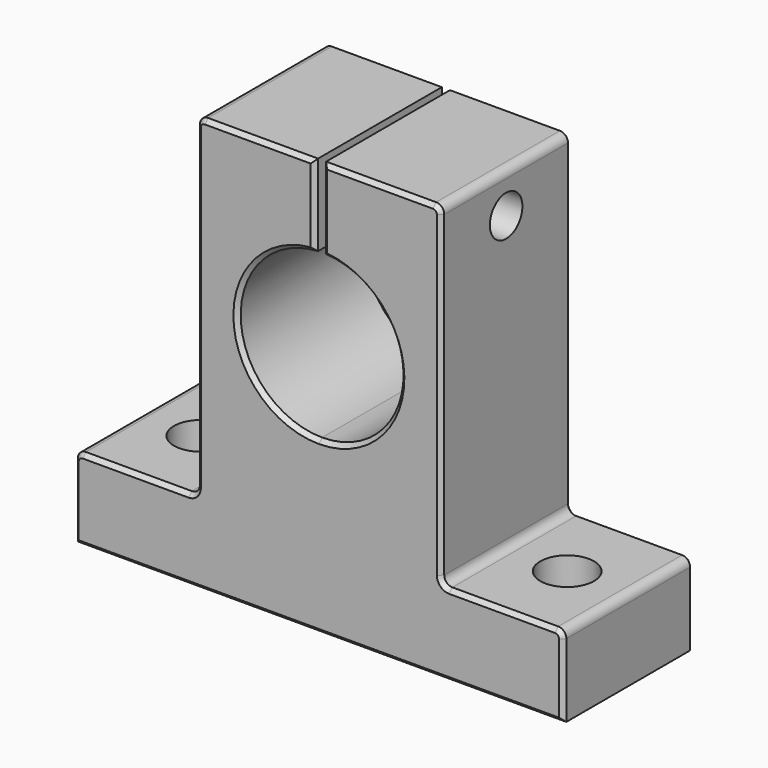
from build123d import *

# Parameters (mm, degrees)
F1_DEPTH    = 10
F3_D        = 6.6
F6_D        = 5
F6_DEPTH    = 22
F6_TIP      = 1.5021515476
F7_R        = 1
F8_C1_SIZE  = 0.5
F8_C2_SIZE  = 0.5
F8_C3_SIZE  = 0.5
F8_C4_SIZE  = 0.5
F8_C5_SIZE  = 0.5
F8_C6_SIZE  = 0.5
F8_C7_SIZE  = 0.5
F8_C8_SIZE  = 0.5
F8_C9_SIZE  = 0.5
F8_C10_SIZE = 0.5
F8_C11_SIZE = 0.5
F8_C12_SIZE = 0.5


with BuildPart() as f1:
    # F0 (on Front) → F1 (new body, symmetric)
    with BuildSketch(Plane.XZ):
        with BuildLine():
            Line((15, 51), (0.5, 51))
            Line((0.5, 51), (0.5, 40.9874921777))
            ThreePointArc((0.5, 40.9874921777), (9.9968725554, 30.7499217894), (0, 21))
            Line((0, 21), (0, 0))
            Line((0, 0), (30, 0))
            Line((30, 0), (30, 10))
            Line((30, 10), (15, 10))
            Line((15, 10), (15, 51))
        make_face()
    extrude(amount=F1_DEPTH, both=True)

    # F3 (through all)
    with Locations(Plane(origin=(0, 0, 0), x_dir=(1, 0, 0), z_dir=(0, 0, -1))):
        with Locations((22.5, 0)):
            Hole(F3_D / 2)

    # F4: F1 across plane


with BuildPart() as f1_1:
    add(f1.part)
    add(f1.part.mirror(Plane.YZ))

    # F6
    with Locations(Plane.YZ.offset(15)):
        with Locations((0, 46)):
            Hole(F6_D / 2, depth=F6_DEPTH)
            with Locations((0, 0, -(F6_DEPTH + F6_TIP / 2))):  # 118° drill point
                Cone(0, F6_D / 2, F6_TIP, mode=Mode.SUBTRACT)

    # F7
    f7_edges = [f1_1.edges().sort_by_distance(p)[0] for p in [
        (15, 0, 10),
        (-15, 0, 10),
        (-30, 0, 10),
        (30, 0, 10),
        (15, 0, 51),
        (-15, 0, 51),
    ]]
    fillet(f7_edges, radius=F7_R)

    # F8: chamfer of 0.5 on 36 edges, made by hand

    # F8_c1
    f8_c1_edges = [f1_1.edges().sort_by_distance(p)[0] for p in [
        (30, 10, 4.5),
        (29.7071067812, 10, 9.7071067812),
        (22.5, 10, 10),
        (15.2928932188, 10, 10.2928932188),
        (15, 10, 30.5),
        (14.7071067812, 10, 50.7071067812),
        (7.25, 10, 51),
    ]]
    chamfer(f8_c1_edges, length=F8_C1_SIZE)

    # F8_c2
    f8_c2_edges = [f1_1.edges().sort_by_distance(p)[0] for p in [
        (-0.25, 10, 0),
    ]]
    chamfer(f8_c2_edges, length=F8_C2_SIZE)

    # F8_c3
    f8_c3_edges = [f1_1.edges().sort_by_distance(p)[0] for p in [
        (-30, 10, 4.75),
        (-29.7071067812, 10, 9.7071067812),
        (-22.5, 10, 10),
        (-15.2928932188, 10, 10.2928932188),
        (-15, 10, 30.5),
        (-14.7071067812, 10, 50.7071067812),
        (-7.25, 10, 51),
    ]]
    chamfer(f8_c3_edges, length=F8_C3_SIZE)

    # F8_c4
    f8_c4_edges = [f1_1.edges().sort_by_distance(p)[0] for p in [
        (0.5, 10, 45.7437460889),
    ]]
    chamfer(f8_c4_edges, length=F8_C4_SIZE)

    # F8_c5
    f8_c5_edges = [f1_1.edges().sort_by_distance(p)[0] for p in [
        (-0.2507065513, 10, 21.0031431827),
    ]]
    chamfer(f8_c5_edges, length=F8_C5_SIZE)

    # F8_c6
    f8_c6_edges = [f1_1.edges().sort_by_distance(p)[0] for p in [
        (-0.5, 10, 45.9940442409),
    ]]
    chamfer(f8_c6_edges, length=F8_C6_SIZE)

    # F8_c7
    f8_c7_edges = [f1_1.edges().sort_by_distance(p)[0] for p in [
        (30, -10, 4.5),
        (29.7071067812, -10, 9.7071067812),
        (22.5, -10, 10),
        (15.2928932188, -10, 10.2928932188),
        (15, -10, 30.5),
        (14.7071067812, -10, 50.7071067812),
        (7.25, -10, 51),
    ]]
    chamfer(f8_c7_edges, length=F8_C7_SIZE)

    # F8_c8
    f8_c8_edges = [f1_1.edges().sort_by_distance(p)[0] for p in [
        (-0.25, -10, 0),
    ]]
    chamfer(f8_c8_edges, length=F8_C8_SIZE)

    # F8_c9
    f8_c9_edges = [f1_1.edges().sort_by_distance(p)[0] for p in [
        (-30, -10, 4.75),
        (-29.7071067812, -10, 9.7071067812),
        (-22.5, -10, 10),
        (-15.2928932188, -10, 10.2928932188),
        (-15, -10, 30.5),
        (-14.7071067812, -10, 50.7071067812),
        (-7.25, -10, 51),
    ]]
    chamfer(f8_c9_edges, length=F8_C9_SIZE)

    # F8_c10
    f8_c10_edges = [f1_1.edges().sort_by_distance(p)[0] for p in [
        (0.5, -10, 45.7437460889),
    ]]
    chamfer(f8_c10_edges, length=F8_C10_SIZE)

    # F8_c11
    f8_c11_edges = [f1_1.edges().sort_by_distance(p)[0] for p in [
        (-0.2507065513, -10, 21.0031431827),
    ]]
    chamfer(f8_c11_edges, length=F8_C11_SIZE)

    # F8_c12
    f8_c12_edges = [f1_1.edges().sort_by_distance(p)[0] for p in [
        (-0.5, -10, 45.9940442409),
    ]]
    chamfer(f8_c12_edges, length=F8_C12_SIZE)


solid = f1_1.part
